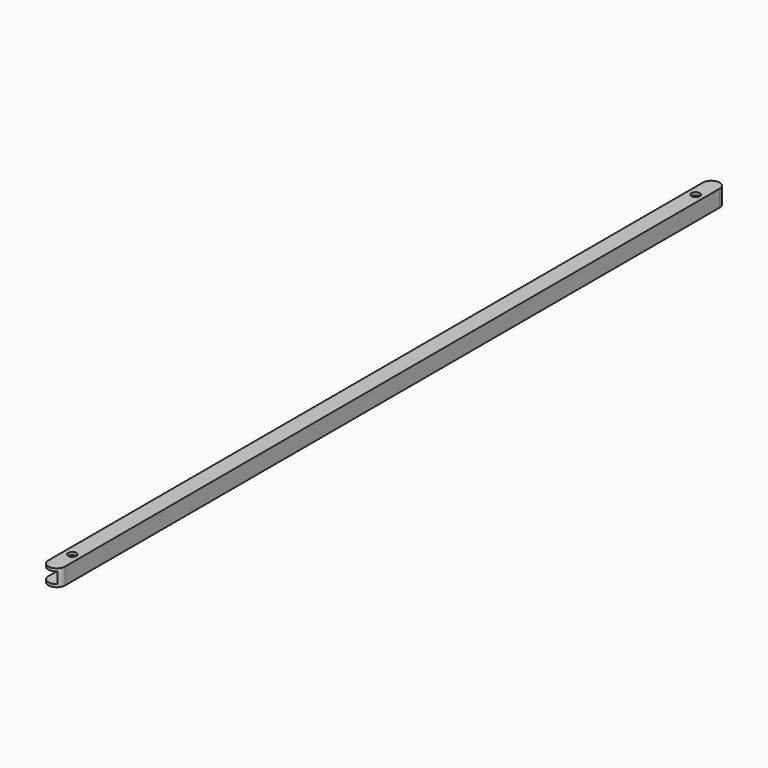
from build123d import *

# Parameters (mm, degrees)
F0_W        = 38.1
F0_H        = 38.1
F0_W_2      = 25.4
F0_H_2      = 25.4
F1_DEPTH    = 952.5
F2_R        = 9.525
F3_DEPTH    = 76.2
F4_W        = 127
F4_H        = 25.4
F5_DEPTH    = 25.4
F6_T1_DEPTH = 133.35
F6_T3_DEPTH = 101.6
F6_T5_DEPTH = 101.6


# Not quite as in the source:
# - a fillet or chamfer that OpenCascade refuses, or shapes differently, is made with other operations: its cross-section is extruded or revolved along the edge and cut away or added


with BuildPart() as f1:
    # F0 (on Front) → F1 (new body, symmetric)
    with BuildSketch(Plane.XZ):
        Rectangle(F0_W, F0_H)
        Rectangle(F0_W_2, F0_H_2, mode=Mode.SUBTRACT)
    extrude(amount=F1_DEPTH, both=True)

    # F2 (on face) → F3 (cut)
    with BuildSketch(Plane.XY.offset(19.05)):
        with Locations((0, -889)):
            Circle(F2_R)
        with Locations((0, 889)):
            Circle(F2_R)
    extrude(amount=-F3_DEPTH, mode=Mode.SUBTRACT)

    # F4 (on Right) → F5 (cut)
    with BuildSketch(Plane.YZ):
        with Locations((901.7, 0)):
            Rectangle(F4_W, F4_H)
        with Locations((-901.7, 0)):
            Rectangle(F4_W, F4_H)
    extrude(amount=-F5_DEPTH, mode=Mode.SUBTRACT)

    # F6: fillet of radius 19.05 on 6 edges, made by hand

    # F6_s2 → F6_t1 (cut)
    with BuildSketch(Plane.XY.offset(-66.675)):
        with BuildLine():
            ThreePointArc((19.05, -933.45), (13.4703841816, -946.9203841816), (0, -952.5))
            Line((0, -952.5), (19.05, -952.5))
            Line((19.05, -952.5), (19.05, -933.45))
        make_face()
        with BuildLine():
            ThreePointArc((19.05, 933.45), (13.4703841816, 946.9203841816), (0, 952.5))
            Line((0, 952.5), (19.05, 952.5))
            Line((19.05, 952.5), (19.05, 933.45))
        make_face()
    extrude(amount=F6_T1_DEPTH, mode=Mode.SUBTRACT)

    # F6_s4 → F6_t3 (cut)
    with BuildSketch(Plane.XY.offset(-34.925)):
        with BuildLine():
            ThreePointArc((-19.05, -933.45), (-13.4703841816, -946.9203841816), (0, -952.5))
            Line((0, -952.5), (-19.05, -952.5))
            Line((-19.05, -952.5), (-19.05, -933.45))
        make_face()
        with BuildLine():
            ThreePointArc((-19.05, 933.45), (-13.4703841816, 946.9203841816), (0, 952.5))
            Line((0, 952.5), (-19.05, 952.5))
            Line((-19.05, 952.5), (-19.05, 933.45))
        make_face()
    extrude(amount=F6_T3_DEPTH, mode=Mode.SUBTRACT)

    # F6_s6 → F6_t5 (cut)
    with BuildSketch(Plane.XY.offset(-66.675)):
        with BuildLine():
            ThreePointArc((-19.05, -933.45), (-13.4703841816, -946.9203841816), (0, -952.5))
            Line((0, -952.5), (-19.05, -952.5))
            Line((-19.05, -952.5), (-19.05, -933.45))
        make_face()
        with BuildLine():
            ThreePointArc((-19.05, 933.45), (-13.4703841816, 946.9203841816), (0, 952.5))
            Line((0, 952.5), (-19.05, 952.5))
            Line((-19.05, 952.5), (-19.05, 933.45))
        make_face()
    extrude(amount=F6_T5_DEPTH, mode=Mode.SUBTRACT)


solid = f1.part
